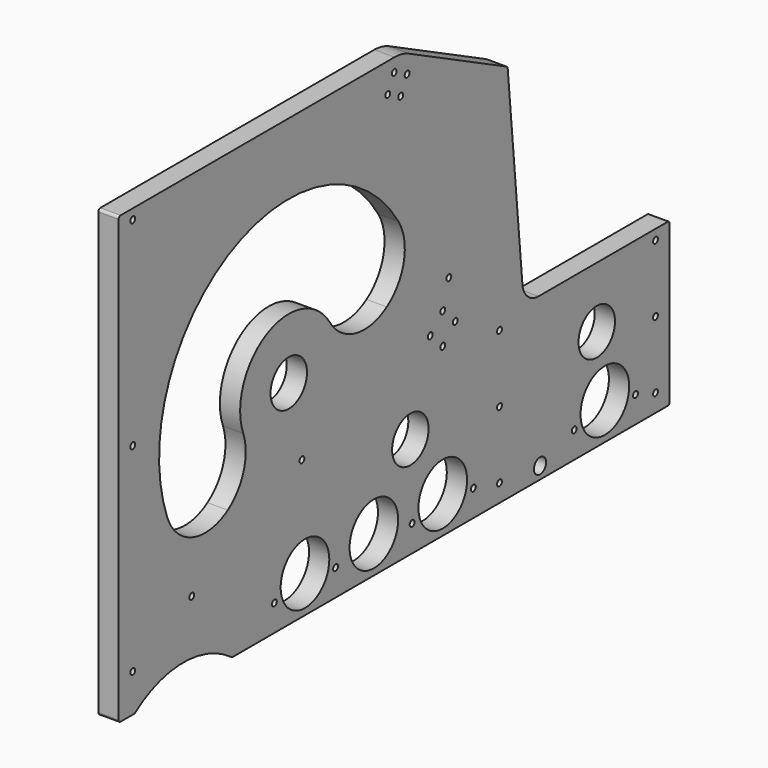
from build123d import *

# Parameters (mm, degrees)
F0_R     = 1.905
F0_R_2   = 14.2875
F0_R_3   = 4.7625
F1_DEPTH = 12.7
F2_R     = 19.05
F3_DEPTH = 12.7
F5_DEPTH = 12.7
F6_R     = 1.905
F7_DEPTH = 12.7
F8_R     = 31.74999
F9_R     = 25.4
F10_R    = 12.7
F11_R    = 1.5875


# Not quite as in the source:
# - a fillet or chamfer is up to 0.001 mm smaller than in the source, because OpenCascade refuses the exact size


with BuildPart() as f1:
    # F0 (on Right) → F1 (new body)
    with BuildSketch(Plane.YZ):
        with BuildLine():
            Line((0, 355.6), (0, 0))
            Line((0, 0), (12.7, 0))
            ThreePointArc((12.7, 0), (50.8, 12.7), (88.9, 0))
            Line((88.9, 0), (431.8, 0))
            Line((431.8, 0), (431.8, 355.6))
            Line((431.8, 355.6), (0, 355.6))
        make_face()
        with Locations((57.329483813, 46.5276031344)):
            Circle(F0_R, mode=Mode.SUBTRACT)
        with Locations((143.6553005282, 86.7819925652)):
            Circle(F0_R, mode=Mode.SUBTRACT)
        with Locations((228.6, 63.5)):
            Circle(F0_R_2, mode=Mode.SUBTRACT)
        with Locations((330.2, 7.62)):
            Circle(F0_R_3, mode=Mode.SUBTRACT)
        with Locations((374.65, 63.5)):
            Circle(F0_R_2, mode=Mode.SUBTRACT)
        with Locations((133.35, 133.35)):
            Circle(F0_R_2, mode=Mode.SUBTRACT)
        with Locations((258.7563894819, 140.4545118063)):
            Circle(F0_R, mode=Mode.SUBTRACT)
    extrude(amount=F1_DEPTH)

    # F2 (on face) → F3 (cut, through all)
    with BuildSketch(Plane.YZ.offset(12.7)):
        with Locations((146.05, 23.05)):
            Circle(F2_R)
        with Locations((254, 23.05)):
            Circle(F2_R)
        with Locations((381, 23.0378)):
            Circle(F2_R)
        with Locations((200.025, 23.05)):
            Circle(F2_R)
    extrude(amount=-F3_DEPTH, mode=Mode.SUBTRACT)

    # F4 (on face) → F5 (cut, through all)
    with BuildSketch(Plane.YZ.offset(12.7)):
        Polygon((431.8, 355.6), (0, 355.6), (0, 279.4), (44.45, 279.4), (222.25, 279.4), (304.8, 238.125), (317.5, 101.6), (431.8, 101.6), (431.8, 247.65), align=None)
        with BuildLine():
            ThreePointArc((231.775, 158.5507812379), (146.2540591137, 234.1272060458), (44.45, 182.5368884968))
            ThreePointArc((44.45, 182.5368884968), (31.75, 133.35), (44.45, 84.1631115032))
            ThreePointArc((44.45, 84.1631115032), (50.9265271613, 73.9451927433), (58.5716384481, 64.5695039011))
            Line((58.5716384481, 64.5695039011), (113.1323420197, 101.0567142305))
            ThreePointArc((113.1323420197, 101.0567142305), (112.1703700265, 165.0207005635), (170.9171066227, 139.7))
            ThreePointArc((170.9171066227, 139.7), (171.3165429182, 136.5361605167), (171.45, 133.35))
            ThreePointArc((171.45, 133.35), (170.2668375807, 123.9289011764), (166.7908344859, 115.0929304409))
            Line((166.7908344859, 115.0929304409), (231.775, 158.5507812379))
        make_face()
    extrude(amount=-F5_DEPTH, mode=Mode.SUBTRACT)

    # F6 (on face) → F7 (cut, through all)
    with BuildSketch(Plane.YZ.offset(12.7)):
        with Locations((420.6875, 11.1125)):
            Circle(F6_R)
        with Locations((420.6875, 53.18125)):
            Circle(F6_R)
        with Locations((420.6875, 95.25)):
            Circle(F6_R)
        with Locations((298.45, 11.1125)):
            Circle(F6_R)
        with Locations((298.45, 95.25)):
            Circle(F6_R)
        with Locations((298.45, 53.18125)):
            Circle(F6_R)
        with Locations((11.1125, 23.8125)):
            Circle(F6_R)
        with Locations((122.05, 16.55)):
            Circle(F6_R)
        with Locations((170.05, 16.55)):
            Circle(F6_R)
        with Locations((230, 16.55)):
            Circle(F6_R)
        with Locations((278, 16.55)):
            Circle(F6_R)
        with Locations((357, 16.5378)):
            Circle(F6_R)
        with Locations((405, 16.5378)):
            Circle(F6_R)
        with Locations((11.1125, 273.05)):
            Circle(F6_R)
        with Locations((11.1125, 148.43125)):
            Circle(F6_R)
        with Locations((215.9725987291, 271.1144663844)):
            Circle(F6_R)
        with Locations((210.9129544728, 260.9951778719)):
            Circle(F6_R)
        with Locations((221.0322429853, 255.9355336156)):
            Circle(F6_R)
        with Locations((226.0918872416, 266.0548221281)):
            Circle(F6_R)
        with Locations((254, 124.079)):
            Circle(F6_R)
        with Locations((244.221, 114.3)):
            Circle(F6_R)
        with Locations((254, 104.521)):
            Circle(F6_R)
        with Locations((263.779, 114.3)):
            Circle(F6_R)
    extrude(amount=-F7_DEPTH, mode=Mode.SUBTRACT)

    # F8 (radius 31.75 in the source; OpenCascade refuses exactly that, so slightly less here)
    f8_edges = [f1.edges().sort_by_distance(p)[0] for p in [
        (6.35, 58.571638, 64.569504),
        (6.35, 113.132342, 101.056714),
        (6.35, 166.790834, 115.09293),
        (6.35, 231.775, 158.550781),
    ]]
    fillet(f8_edges, radius=F8_R)

    # F9
    f9_edges = [f1.edges().sort_by_distance(p)[0] for p in [
        (6.35, 222.25, 279.4),
    ]]
    fillet(f9_edges, radius=F9_R)

    # F10
    f10_edges = [f1.edges().sort_by_distance(p)[0] for p in [
        (6.35, 317.5, 101.6),
    ]]
    fillet(f10_edges, radius=F10_R)

    # F11
    f11_edges = [f1.edges().sort_by_distance(p)[0] for p in [
        (6.35, 431.8, 101.6),
        (6.35, 431.8, 0),
        (6.35, 0, 0),
        (6.35, 12.7, 0),
        (6.35, 88.9, 0),
        (6.35, 0, 279.4),
        (6.35, 304.8, 238.125),
    ]]
    fillet(f11_edges, radius=F11_R)


solid = f1.part
